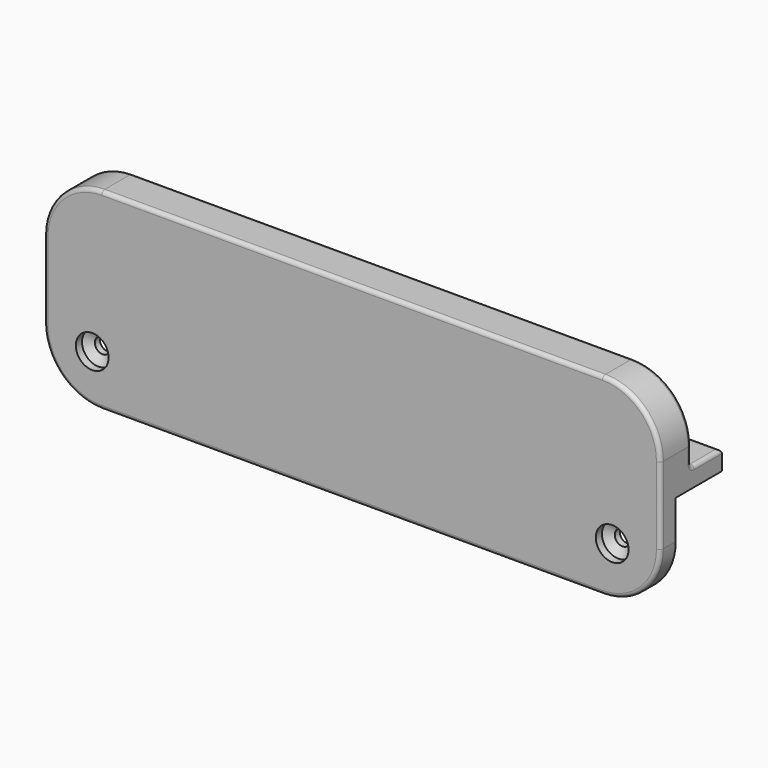
from build123d import *

# Parameters (mm, degrees)
F0_W     = 160
F0_H     = 5
F1_DEPTH = 25
F0_H_2   = 10
F2_DEPTH = 5
F3_DEPTH = 25
F4_R     = 2
F5_DEPTH = 5
F6_D     = 8.5
F6_DEPTH = 2
F6_TIP   = 2.5536576309
F7_R     = 15
F8_R     = 1


with BuildPart() as f1:
    # F0 (on Top) → F1 (new body)
    with BuildSketch(Plane.XY):
        with Locations((80, 2.5)):
            Rectangle(F0_W, F0_H)
        with Locations((80, 7.5)):
            Rectangle(F0_W, F0_H)
    extrude(amount=F1_DEPTH)

    # F0 (on Top) → F2 (join)
    with BuildSketch(Plane.XY):
        with Locations((80, 15)):
            Rectangle(F0_W, F0_H_2)
    extrude(amount=F2_DEPTH)

    # F0 (on Top) → F3 (join)
    with BuildSketch(Plane.XY):
        with Locations((80, 2.5)):
            Rectangle(F0_W, F0_H)
    extrude(amount=-F3_DEPTH)

    # F4 (on face) → F5 (cut, through all)
    with BuildSketch(Plane.XZ):
        with Locations((12.5, -12.5)):
            Circle(F4_R)
        with Locations((147.5, -12.5)):
            Circle(F4_R)
    extrude(amount=-F5_DEPTH, mode=Mode.SUBTRACT)

    # F6
    with Locations(Plane.XZ):
        with Locations((12.5, -12.5), (147.5, -12.5)):
            Hole(F6_D / 2, depth=F6_DEPTH)
            with Locations((0, 0, -(F6_DEPTH + F6_TIP / 2))):  # 118° drill point
                Cone(0, F6_D / 2, F6_TIP, mode=Mode.SUBTRACT)

    # F7
    f7_edges = [f1.edges().sort_by_distance(p)[0] for p in [
        (160, 2.5, -25),
        (0, 2.5, -25),
        (160, 5, 25),
        (0, 5, 25),
    ]]
    fillet(f7_edges, radius=F7_R)

    # F8
    f8_edges = [f1.edges().sort_by_distance(p)[0] for p in [
        (0, 10, 7.5),
        (4.393398, 10, 20.606602),
        (80, 10, 5),
        (80, 10, 25),
        (160, 10, 7.5),
        (155.606602, 10, 20.606602),
        (80, 0, 25),
        (80, 20, 5),
        (0, 0, 0),
        (4.393398, 0, 20.606602),
        (4.393398, 0, -20.606602),
        (80, 0, -25),
        (155.606602, 0, 20.606602),
        (155.606602, 0, -20.606602),
        (160, 0, 0),
        (0, 15, 5),
        (160, 15, 5),
    ]]
    fillet(f8_edges, radius=F8_R)


solid = f1.part
